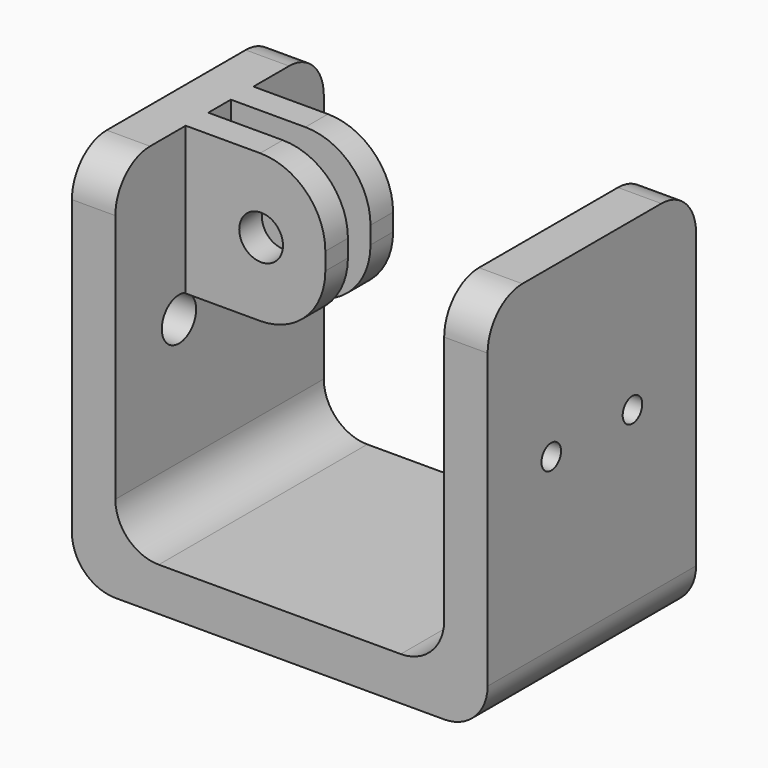
from build123d import *

# Parameters (mm, degrees)
F1_DEPTH  = 30.48
F2_R      = 1.42875
F3_DEPTH  = 67.945
F4_R      = 5.08
F5_R      = 5.08
F6_R      = 5.08
F7_SIZE   = 0.98552
F8_R      = 2.50825
F9_DEPTH  = 18.161
F10_W     = 3.302
F10_H     = 17.272
F11_DEPTH = 16.3322
F12_R     = 5.08
F13_R     = 7.62
F14_R     = 7.62
F16_DEPTH = 25.4


# Not quite as in the source:
# - a feature names something its author has since deleted; it is built from what else it names


with BuildPart() as f1:
    # F0 (on Front) → F1 (new body)
    with BuildSketch(Plane.XZ):
        Polygon((-20.2290668074, 29.0888086691), (-25.3090668074, 29.0888086691), (-25.3090668074, -15.3611913309), (23.3149106546, -15.3611913309), (23.3149106546, 29.0888086691), (18.2349106546, 29.0888086691), (18.2349106546, -10.2811913309), (-20.2290668074, -10.2811913309), align=None)
    extrude(amount=F1_DEPTH)

    # F2 (on face) → F3 (cut)
    with BuildSketch(Plane.YZ.offset(23.3149106546)):
        with Locations((-21.17725, 9.5689086691)):
            Circle(F2_R)
        with BuildLine():
            ThreePointArc((-7.874, 9.5689086691), (-9.30275, 10.9976586691), (-10.7315, 9.5689086691))
            ThreePointArc((-10.7315, 9.5689086691), (-9.30275, 8.1401586691), (-7.874, 9.5689086691))
        make_face()
    extrude(amount=-F3_DEPTH, mode=Mode.SUBTRACT)

    # F4
    f4_edges = [f1.edges().sort_by_distance(p)[0] for p in [
        (20.774911, 0, 29.088809),
        (20.774911, -30.48, 29.088809),
    ]]
    fillet(f4_edges, radius=F4_R)

    # F5
    f5_edges = [f1.edges().sort_by_distance(p)[0] for p in [
        (23.314911, -15.24, -15.361191),
        (18.234911, -15.24, -10.281191),
    ]]
    fillet(f5_edges, radius=F5_R)

    # F6
    f6_edges = [f1.edges().sort_by_distance(p)[0] for p in [
        (-20.229067, -15.24, -10.281191),
        (-25.309067, -15.24, -15.361191),
    ]]
    fillet(f6_edges, radius=F6_R)

    # F7
    f7_edges = [f1.edges().sort_by_distance(p)[0] for p in [
        (18.234911, -7.874, 9.568909),
        (18.234911, -22.606, 9.568909),
    ]]
    chamfer(f7_edges, length=F7_SIZE)

    # F8 (on face) → F9 (cut)
    with BuildSketch(Plane(origin=(-25.3090668074, 0, 0), x_dir=(0, -1, 0), z_dir=(-1, 0, 0))):
        with Locations((21.17725, 9.5689086691)):
            Circle(F8_R)
        with Locations((9.30275, 9.5689086691)):
            Circle(F8_R)
    extrude(amount=-F9_DEPTH, mode=Mode.SUBTRACT)

    # F10 (on face) → F11 (join)
    with BuildSketch(Plane.YZ.offset(-20.2290668074)):
        with Locations((-11.938, 20.4528086691)):
            Rectangle(F10_W, F10_H)
        with Locations((-18.542, 20.4528086691)):
            Rectangle(F10_W, F10_H)
    extrude(amount=F11_DEPTH)

    # F12
    f12_edges = [f1.edges().sort_by_distance(p)[0] for p in [
        (-22.769067, 0, 29.088809),
        (-22.769067, -30.48, 29.088809),
    ]]
    fillet(f12_edges, radius=F12_R)

    # F13
    f13_edges = [f1.edges().sort_by_distance(p)[0] for p in [
        (-3.896867, -11.938, 29.088809),
        (-3.896867, -11.938, 11.816809),
    ]]
    fillet(f13_edges, radius=F13_R)

    # F14
    f14_edges = [f1.edges().sort_by_distance(p)[0] for p in [
        (-3.896867, -18.542, 29.088809),
        (-3.896867, -18.542, 11.816809),
    ]]
    fillet(f14_edges, radius=F14_R)

    # F15 (on face) → F16 (cut)
    with BuildSketch(Plane(origin=(0, -10.287, 0), x_dir=(-1, 0, 0), z_dir=(0, 1, 0))):
        with BuildLine():
            ThreePointArc((8.8498668074, 20.4528086691), (11.4089168074, 17.8937586691), (13.9679668074, 20.4528086691))
            ThreePointArc((13.9679668074, 20.4528086691), (11.4089168074, 23.0118586691), (8.8498668074, 20.4528086691))
        make_face()
    extrude(amount=-F16_DEPTH, mode=Mode.SUBTRACT)


solid = f1.part
